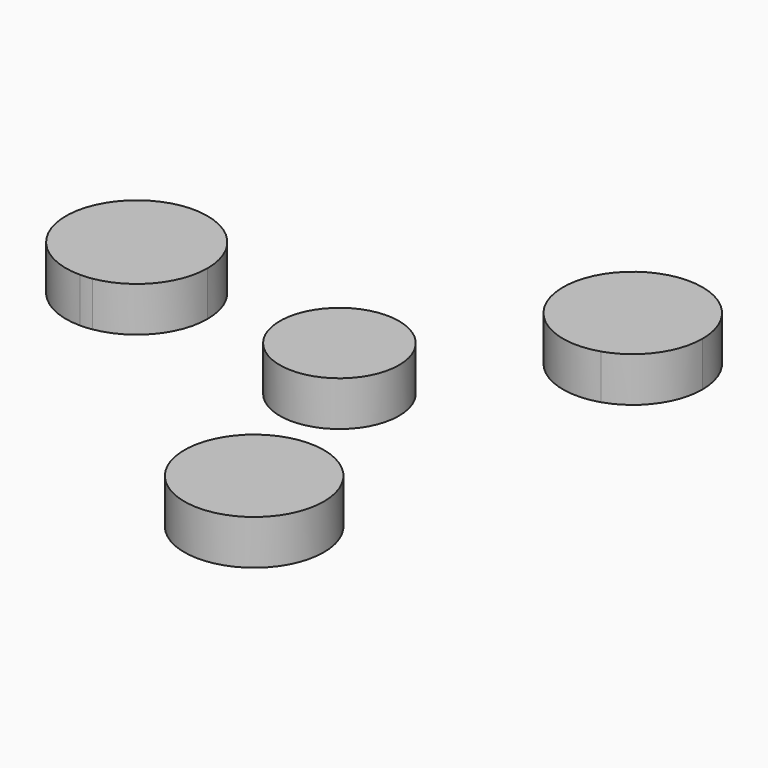
from build123d import *

# Parameters (mm, degrees)
F0_R     = 33.3045819347
F1_DEPTH = 25.4
F0_R_2   = 33.8985173745


with BuildPart() as f1:
    # F0 (on Top) → F1 (new body)
    with BuildSketch(Plane.XY):
        with BuildLine():
            ThreePointArc((10.1881658678, -117.7966108428), (46.3861106689, -163.3243326291), (89.0427784966, -123.7835517983))
            ThreePointArc((89.0427784966, -123.7835517983), (52.3902824548, -84.2427709675), (10.1881658678, -117.7966108428))
        make_face()
        with Locations((49.3881965618, -123.7835517983)):
            Circle(F0_R, mode=Mode.SUBTRACT)
        with Locations((49.3881965618, -123.7835517983)):
            Circle(F0_R)
    extrude(amount=F1_DEPTH)


with BuildPart() as f1b:
    # F0 (on Top) → F1, piece 2 (new body)
    with BuildSketch(Plane.XY):
        with BuildLine():
            ThreePointArc((94.9610891571, 65.6953507789), (114.8894087237, 80.085805582), (122.5079874693, 103.4563076751))
            ThreePointArc((122.5079874693, 103.4563076751), (50.8174023454, 126.8268097682), (94.9610891571, 65.6953507789))
        make_face()
        with Locations((82.8534055346, 103.4563076751)):
            Circle(F0_R, mode=Mode.SUBTRACT)
        with Locations((82.8534055346, 103.4563076751)):
            Circle(F0_R)
    extrude(amount=F1_DEPTH)


with BuildPart() as f1c:
    # F0 (on Top) → F1, piece 3 (new body)
    with BuildSketch(Plane.XY):
        with BuildLine():
            ThreePointArc((-131.653085351, -21.1727726474), (-128.3691135331, -20.8615140587), (-125.0784078119, -20.6321482679))
            ThreePointArc((-125.0784078119, -20.6321482679), (-100.9564717429, -6.9561792095), (-91.4045679764, 19.0757447272))
            ThreePointArc((-91.4045679764, 19.0757447272), (-95.0960352936, 35.9139525283), (-105.4932977209, 49.6634654987))
            ThreePointArc((-105.4932977209, 49.6634654987), (-169.4092342659, 33.0190718037), (-131.653085351, -21.1727726474))
        make_face()
        with Locations((-131.653085351, 19.0757447272)):
            Circle(F0_R_2, mode=Mode.SUBTRACT)
        with Locations((-131.653085351, 19.0757447272)):
            Circle(F0_R_2)
        with BuildLine():
            ThreePointArc((-131.653085351, -21.1727726474), (-128.3546516521, -21.0373888575), (-125.0784078119, -20.6321482679))
            ThreePointArc((-125.0784078119, -20.6321482679), (-128.3691135331, -20.8615140587), (-131.653085351, -21.1727726474))
        make_face()
    extrude(amount=F1_DEPTH)


with BuildPart() as f1d:
    # F0 (on Top) → F1, piece 4 (new body)
    with BuildSketch(Plane.XY):
        with Locations((-0.7478448097, -0.4991076421)):
            Circle(F0_R_2)
    extrude(amount=F1_DEPTH)


solid = Compound([f1.part, f1b.part, f1c.part, f1d.part])
